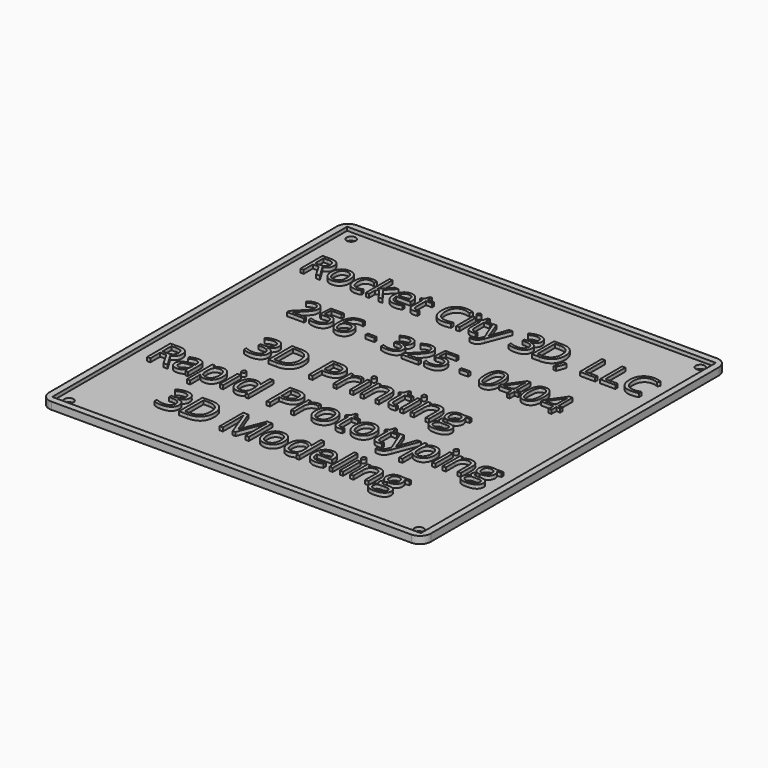
from build123d import *

# Parameters (mm, degrees)
F0_W           = 266.7
F0_H           = 266.7
F1_DEPTH       = 2.54
F2_W           = 266.7
F2_H           = 266.7
F2_W_2         = 257.5559914112
F2_H_2         = 257.5559914112
F3_DEPTH       = 2.54
F4_TEXT_SIZE   = 27.0895312939
F4_TEXT_SIZE_2 = 25.5881797385
F4_TEXT_SIZE_3 = 28.6946988982
F5_DEPTH       = 2.54
F6_R           = 7.62
F7_R           = 3.175
F8_DEPTH       = 2.541


# Not quite as in the source:
# - Text() gives the source's letters only with a copy of the font that has no kerning and outlines rounded to 1/6400 em; it was checked with that copy


with BuildPart() as f1:
    # F0 (on Top) → F1 (new body)
    with BuildSketch(Plane.XY):
        Rectangle(F0_W, F0_H)
    extrude(amount=F1_DEPTH)

    # F2 (on face) → F3 (join)
    with BuildSketch(Plane.XY.offset(2.54)):
        Rectangle(F2_W, F2_H)
        Rectangle(F2_W_2, F2_H_2, mode=Mode.SUBTRACT)
    extrude(amount=F3_DEPTH)

    # F4 (on face) → F5 (join)
    with BuildSketch(Plane.XY.offset(2.54)):
        with Locations((-120.3884847787, 74.1992416473)):
            Text('Rocket City 3D, LLC', F4_TEXT_SIZE, font='Open Sans', text_align=(TextAlign.LEFT, TextAlign.BOTTOM))
        with Locations((-92.6696434617, 29.4447429478)):
            Text('256 - 325 - 0404', F4_TEXT_SIZE_2, font='Open Sans', text_align=(TextAlign.LEFT, TextAlign.BOTTOM))
        with Locations((-83.3693091659, -20.6601832067)):
            Text('3D Printing', F4_TEXT_SIZE_3, font='Open Sans', text_align=(TextAlign.LEFT, TextAlign.BOTTOM))
        with Locations((-120.65, -59.6849737082)):
            Text('Rapid Prototyping', F4_TEXT_SIZE_3, font='Open Sans', text_align=(TextAlign.LEFT, TextAlign.BOTTOM))
        with Locations((-83.3693091659, -98.7097642097)):
            Text('3D Modeling', F4_TEXT_SIZE_3, font='Open Sans', text_align=(TextAlign.LEFT, TextAlign.BOTTOM))
    extrude(amount=F5_DEPTH)

    # F6
    f6_edges = [f1.edges().sort_by_distance(p)[0] for p in [
        (-133.35, 133.35, 2.54),
        (133.35, 133.35, 2.54),
        (133.35, -133.35, 2.54),
        (-133.35, -133.35, 2.54),
    ]]
    fillet(f6_edges, radius=F6_R)

    # F7 (on face) → F8 (cut, through all)
    with BuildSketch(Plane.XY.offset(2.54)):
        with Locations((-120.9053245205, 122.4279957056)):
            Circle(F7_R)
        with Locations((122.4708333611, 123.1687739491)):
            Circle(F7_R)
        with Locations((-121.900969754, -122.6880414054)):
            Circle(F7_R)
        with Locations((122.4279957056, -122.4279957056)):
            Circle(F7_R)
    extrude(amount=-F8_DEPTH, mode=Mode.SUBTRACT)


solid = f1.part
